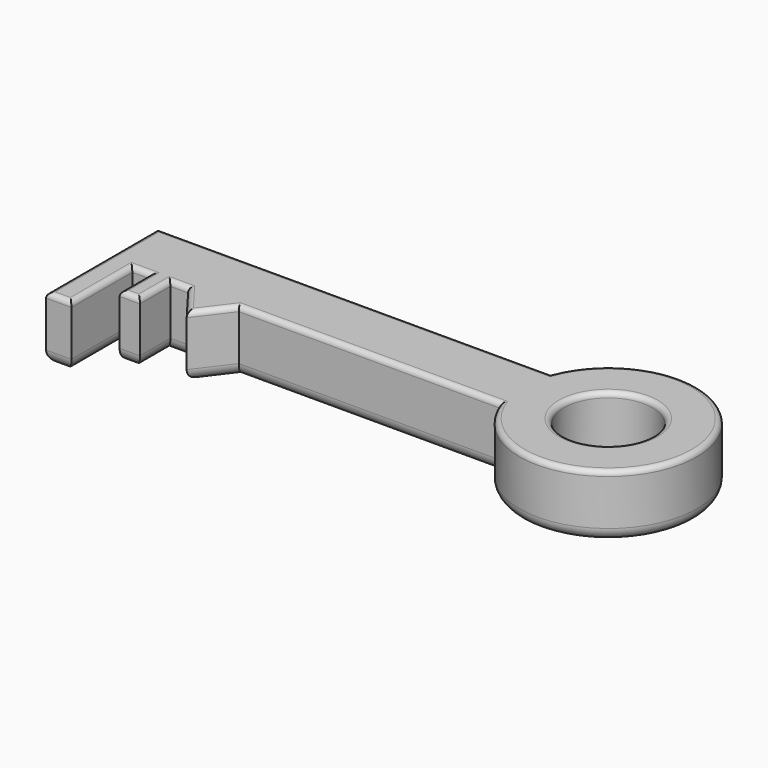
from build123d import *

# Parameters (mm, degrees)
F0_R     = 17.5
F0_W     = 10
F0_H     = 30
F0_W_2   = 8
F0_H_2   = 15
F1_DEPTH = 25
F2_R     = 2
F3_R     = 4.99999


# Not quite as in the source:
# - a fillet or chamfer is up to 0.001 mm smaller than in the source, because OpenCascade refuses the exact size


with BuildPart() as f1:
    # F0 (on Top) → F1 (new body)
    with BuildSketch(Plane.XY):
        with BuildLine():
            Line((86.0379100244, 2.0564989746), (-68.9620899756, 2.0564989746))
            Line((-68.9620899756, 2.0564989746), (-68.9620899756, -22.9435010254))
            Line((-68.9620899756, -22.9435010254), (-58.9620899756, -22.9435010254))
            Line((-58.9620899756, -22.9435010254), (-51.9620899756, -22.9435010254))
            Line((-51.9620899756, -22.9435010254), (-43.9620899756, -22.9435010254))
            Line((-43.9620899756, -22.9435010254), (-36.9620899756, -22.9435010254))
            Line((-36.9620899756, -22.9435010254), (-16.9620899756, -22.9435010254))
            Line((-16.9620899756, -22.9435010254), (86.0379100244, -22.9435010254))
            ThreePointArc((86.0379100244, -22.9435010254), (153.7296521009, -10.4435010254), (86.0379100244, 2.0564989746))
        make_face()
        with Locations((118.7296521009, -10.4435010254)):
            Circle(F0_R, mode=Mode.SUBTRACT)
        with Locations((-63.9620899756, -37.9435010254)):
            Rectangle(F0_W, F0_H)
        with Locations((-47.9620899756, -30.4435010254)):
            Rectangle(F0_W_2, F0_H_2)
        Polygon((-26.9620899756, -36.1344755535), (-16.9620899756, -22.9435010254), (-36.9620899756, -22.9435010254), align=None)
    extrude(amount=F1_DEPTH)

    # F2
    f2_edges = [f1.edges().sort_by_distance(p)[0] for p in [
        (8.53791, 2.056499, 25),
        (34.53791, -22.943501, 25),
        (-21.96209, -29.538988, 25),
        (-31.96209, -29.538988, 25),
        (-40.46209, -22.943501, 25),
        (-43.96209, -30.443501, 25),
        (-47.96209, -37.943501, 25),
        (-55.46209, -22.943501, 25),
        (-51.96209, -30.443501, 25),
        (-58.96209, -37.943501, 25),
        (-63.96209, -52.943501, 25),
        (-68.96209, -25.443501, 25),
        (153.729652, -10.443501, 25),
        (101.229652, -10.443501, 25),
    ]]
    fillet(f2_edges, radius=F2_R)

    # F3 (radius 5 in the source; OpenCascade refuses exactly that, so slightly less here)
    f3_edges = [f1.edges().sort_by_distance(p)[0] for p in [
        (-21.96209, -29.538988, 0),
        (-31.96209, -29.538988, 0),
        (34.53791, -22.943501, 0),
        (8.53791, 2.056499, 0),
        (-43.96209, -30.443501, 0),
        (-47.96209, -37.943501, 0),
        (-40.46209, -22.943501, 0),
        (-55.46209, -22.943501, 0),
        (-58.96209, -37.943501, 0),
        (-68.96209, -25.443501, 0),
        (-63.96209, -52.943501, 0),
        (153.729652, -10.443501, 0),
        (101.229652, -10.443501, 0),
    ]]
    fillet(f3_edges, radius=F3_R)


solid = f1.part
